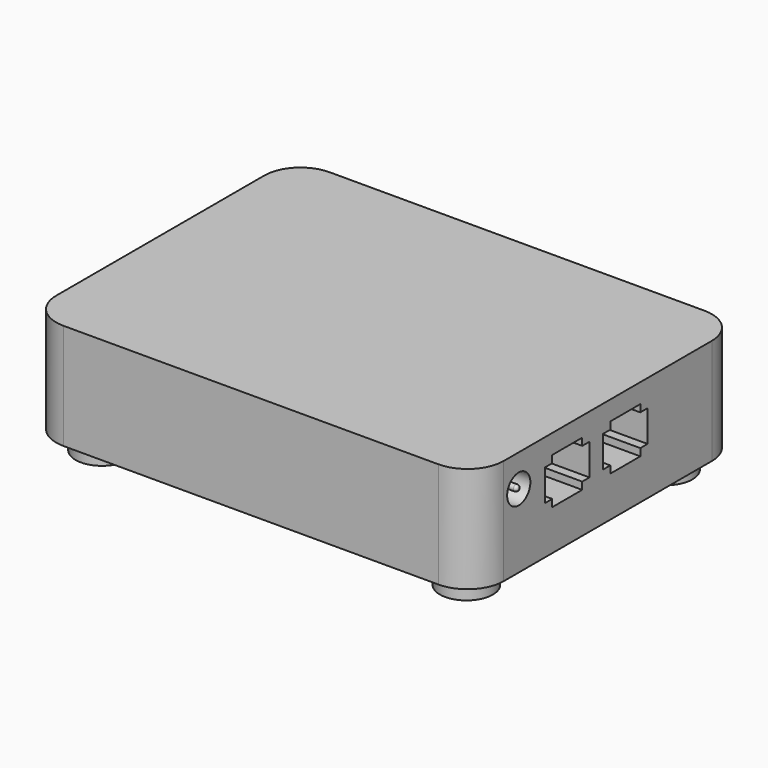
from build123d import *

# Parameters (mm, degrees)
F0_W      = 93.98
F0_H      = 69.85
F1_DEPTH  = 22.225
F2_W      = 10.31875
F2_H      = 15.875
F3_DEPTH  = 4.7625
F4_R      = 5.08
F5_R      = 5.55625
F6_DEPTH  = 3.96875
F8_R      = 7.62
F9_W      = 7.874
F9_H      = 1.524
F9_W_2    = 1.905
F9_H_2    = 6.604
F10_DEPTH = 10.668
F11_DEPTH = 10.668
F9_R      = 3.048
F12_DEPTH = 10.668
F13_R     = 0.635
F14_DEPTH = 10.668
F15_R     = 0.6096
F7_R      = 3.96875
F16_DEPTH = 4.7625


with BuildPart() as f1:
    # F0 (on Top) → F1 (new body)
    with BuildSketch(Plane.XY):
        Rectangle(F0_W, F0_H)
    extrude(amount=F1_DEPTH)

    # F2 (on face) → F3 (join)
    with BuildSketch(Plane(origin=(0, 0, 0), x_dir=(1, 0, 0), z_dir=(0, 0, -1))):
        with Locations((-35.480625, 0)):
            Rectangle(F2_W, F2_H)
        with Locations((35.480625, 0)):
            Rectangle(F2_W, F2_H)
    extrude(amount=F3_DEPTH)

    # F4
    f4_edges = [f1.edges().sort_by_distance(p)[0] for p in [
        (-30.32125, -7.9375, -2.38125),
        (-40.64, -7.9375, -2.38125),
        (30.32125, -7.9375, -2.38125),
        (40.64, -7.9375, -2.38125),
        (40.64, 7.9375, -2.38125),
        (30.32125, 7.9375, -2.38125),
        (-30.32125, 7.9375, -2.38125),
        (-40.64, 7.9375, -2.38125),
    ]]
    fillet(f4_edges, radius=F4_R)

    # F5 (on face) → F6 (join)
    with BuildSketch(Plane(origin=(0, 0, 0), x_dir=(1, 0, 0), z_dir=(0, 0, -1))):
        with Locations((38.25875, 26.19375)):
            Circle(F5_R)
        with Locations((-38.25875, -26.19375)):
            Circle(F5_R)
        with Locations((38.25875, -26.19375)):
            Circle(F5_R)
        with Locations((-38.25875, 26.19375)):
            Circle(F5_R)
    extrude(amount=F6_DEPTH)

    # F8
    f8_edges = [f1.edges().sort_by_distance(p)[0] for p in [
        (-46.99, -34.925, 11.1125),
        (46.99, -34.925, 11.1125),
        (46.99, 34.925, 11.1125),
        (-46.99, 34.925, 11.1125),
    ]]
    fillet(f8_edges, radius=F8_R)

    # F9 (on face) → F10 (cut)
    with BuildSketch(Plane.YZ.offset(46.99)):
        with Locations((-10.643445003, 17.399)):
            Rectangle(F9_W, F9_H)
        with Locations((-5.753945003, 13.335)):
            Rectangle(F9_W_2, F9_H_2)
        with Locations((-10.643445003, 13.335)):
            Rectangle(F9_W, F9_H_2)
        with Locations((-15.532945003, 13.335)):
            Rectangle(F9_W_2, F9_H_2)
        with Locations((-10.643445003, 9.271)):
            Rectangle(F9_W, F9_H)
    extrude(amount=-F10_DEPTH, mode=Mode.SUBTRACT)

    # F9 (on face) → F11 (cut)
    with BuildSketch(Plane.YZ.offset(46.99)):
        with Locations((-0.292945003, 13.335)):
            Rectangle(F9_W_2, F9_H_2)
        with Locations((4.596554997, 17.399)):
            Rectangle(F9_W, F9_H)
        with Locations((4.596554997, 9.271)):
            Rectangle(F9_W, F9_H)
        with Locations((4.596554997, 13.335)):
            Rectangle(F9_W, F9_H_2)
        with Locations((9.486054997, 13.335)):
            Rectangle(F9_W_2, F9_H_2)
    extrude(amount=-F11_DEPTH, mode=Mode.SUBTRACT)

    # F9 (on face) → F12 (cut)
    with BuildSketch(Plane.YZ.offset(46.99)):
        with Locations((-23.368, 15.4551044106)):
            Circle(F9_R)
    extrude(amount=-F12_DEPTH, mode=Mode.SUBTRACT)

    # F13 (on face) → F14 (join)
    with BuildSketch(Plane.YZ.offset(36.322)):
        with Locations((-23.368, 15.4551044106)):
            Circle(F13_R)
    extrude(amount=F14_DEPTH)

    # F15
    f15_edges = [f1.edges().sort_by_distance(p)[0] for p in [
        (46.99, -24.003, 15.455104),
    ]]
    fillet(f15_edges, radius=F15_R)

    # F7 (on face) → F16 (cut)
    with BuildSketch(Plane(origin=(0, 0, -4.7625), x_dir=(1, 0, 0), z_dir=(0, 0, -1))):
        with Locations((-35.40125, 2.8575)):
            Circle(F7_R)
        with Locations((35.40125, 2.8575)):
            Circle(F7_R)
    extrude(amount=-F16_DEPTH, mode=Mode.SUBTRACT)


solid = f1.part
